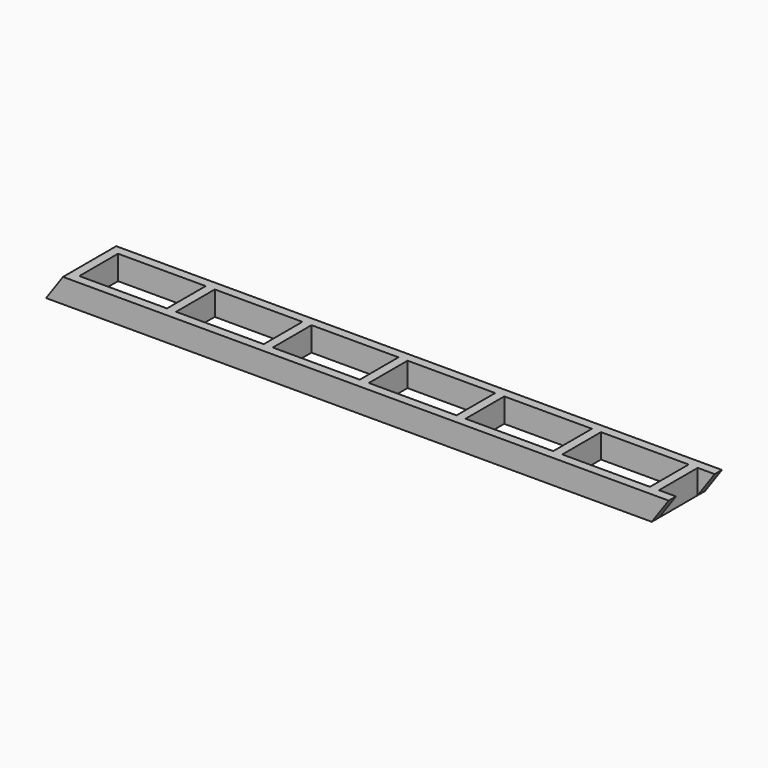
from build123d import *

# Parameters (mm, degrees)
F1_DEPTH = 38.1
F2_W     = 38.1
F2_H     = 101.6
F3_DEPTH = 203.2
F4_W     = 38.1
F4_H     = 101.6
F5_DEPTH = 38.1


# Not quite as in the source:
# - a feature names something its author has since deleted; it is built from what else it names


with BuildPart() as f1:
    # F0 (on Front) → F1 (new body)
    with BuildSketch(Plane.XZ):
        Polygon((71.1410858821, 101.6), (0, 0), (2544.7625, 0), (2615.9035858821, 101.6), align=None)
    extrude(amount=F1_DEPTH)

    # F2 (on face) → F3 (join)
    with BuildSketch(Plane.XZ.offset(38.1)):
        with Locations((90.1910858821, 50.8)):
            Rectangle(F2_W, F2_H)
        with Locations((496.5910858821, 50.8)):
            Rectangle(F2_W, F2_H)
        with Locations((902.9910858821, 50.8)):
            Rectangle(F2_W, F2_H)
        with Locations((1306.5125, 50.8)):
            Rectangle(F2_W, F2_H)
        with Locations((1712.9125, 50.8)):
            Rectangle(F2_W, F2_H)
        with Locations((2119.3125, 50.8)):
            Rectangle(F2_W, F2_H)
        with Locations((2525.7125, 50.8)):
            Rectangle(F2_W, F2_H)
    extrude(amount=F3_DEPTH)

    # F4 (on face) → F5 (join)
    with BuildSketch(Plane.XZ.offset(241.3)):
        Polygon((2615.9035858821, 101.6), (109.2410858821, 101.6), (109.2410858821, 0), (2544.7625, 0), align=None)
        with Locations((90.1910858821, 50.8)):
            Rectangle(F4_W, F4_H)
        Polygon((71.1410858821, 101.6), (0, 0), (71.1410858821, 0), align=None)
    extrude(amount=F5_DEPTH)


solid = f1.part
